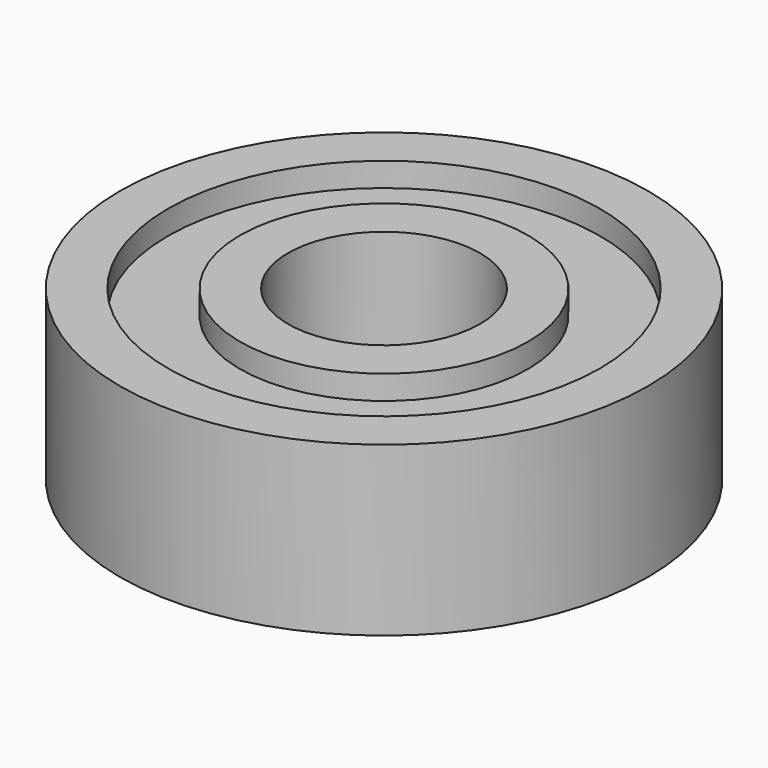
from build123d import *

# Parameters (mm, degrees)
F0_R     = 11
F0_R_2   = 4
F1_DEPTH = 7
F2_T     = -2
F3_DEPTH = 4
F4_T     = 2
F5_DEPTH = 3


# Not quite as in the source:
# - a shell that OpenCascade refuses in one call is made with other operations: the cavity is built on its own and cut out


with BuildPart() as f1:
    # F0 (on Top) → F1 (new body)
    with BuildSketch(Plane.XY):
        Circle(F0_R)
        Circle(F0_R_2, mode=Mode.SUBTRACT)
    extrude(amount=F1_DEPTH)

    # F2
    f2_openings = [f1.faces().sort_by_distance(p)[0] for p in [
        (-10.688873, 0, 7),
    ]]
    offset(amount=F2_T, openings=f2_openings)

    # F3 (add): a face of the model
    f3_faces = [f1.faces().sort_by_distance(p)[0] for p in [
        (-8.7454415588, 0, 2),
    ]]
    extrude(f3_faces, amount=F3_DEPTH)

    # F4: shell of thickness 2, made by hand


with BuildPart() as f4_core1:
    # F4_t2: copy of F1
    add(f1.part)

    # the walls: a layer under each face that stays
    f4_faces = [f4_core1.faces().sort_by_distance(p)[0] for p in [
        (-11, 0, 3.5),
        (-7.3333333333, -7.3333333333, 7),
        (-4, 0, 3.5),
        (-9, 0, 6.5),
        (-4, -4, 7),
        (-6, -6, 6),
        (-6, 0, 6.5),
    ]]
    thicken(f4_faces, amount=-F4_T, mode=Mode.SUBTRACT)

    # F4_s3 → F4_t4 (revolve, cut)
    with BuildSketch(Plane.XZ):
        Polygon((8.98, 6.02), (11, 6), (11, 4), (9, 4), align=None)
    revolve(axis=Axis((0, 0, 6), (0, 0, -1)), mode=Mode.SUBTRACT)

    # F4_s5 → F4_t6 (revolve, cut)
    with BuildSketch(Plane.XZ):
        Polygon((6.02, 6.02), (6, 4), (4, 4), (4, 6), align=None)
    revolve(axis=Axis((0, 0, 6), (0, 0, -1)), mode=Mode.SUBTRACT)


with BuildPart() as f1_1:
    add(f1.part)

    # what is left inside the walls is the cavity
    f4_cavity = [f4_core1.part.solids().sort_by_distance(p)[0] for p in [
        (-8.98, 0, 2.666667),
    ]]
    add(f4_cavity, mode=Mode.SUBTRACT)

    # F5 (add): a face of the model
    f5_faces = [f1_1.faces().sort_by_distance(p)[0] for p in [
        (-8.7454415588, 0, 4),
    ]]
    extrude(f5_faces, amount=F5_DEPTH)


solid = f1_1.part
